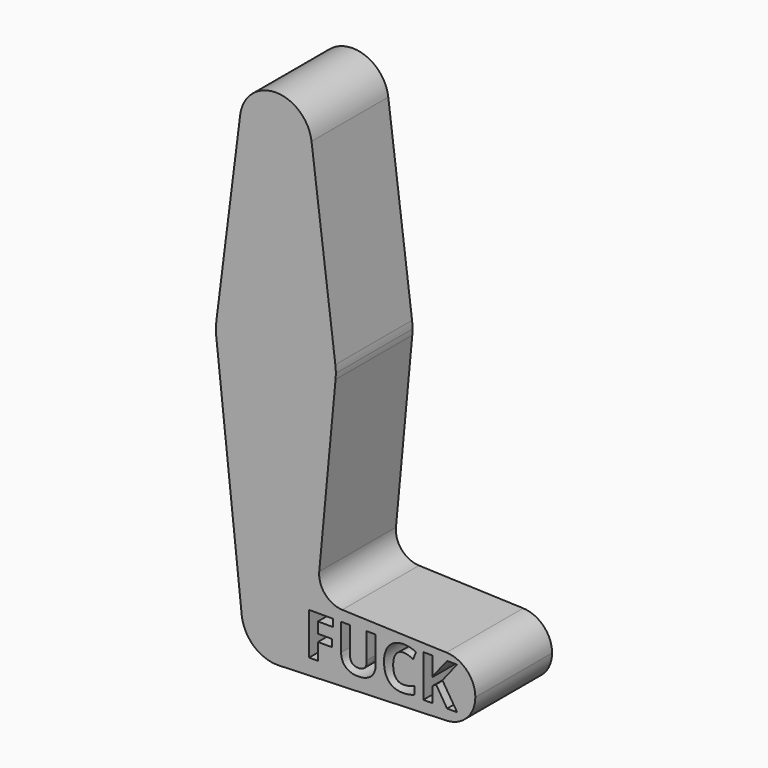
from build123d import *

# Parameters (mm, degrees)
F1_DEPTH     = 25.4
F2_TEXT_SIZE = 15.5810214993
F3_DEPTH     = 25.4


# Not quite as in the source:
# - Text() gives the source's letters only with a copy of the font that has no kerning and outlines rounded to 1/6400 em; it was checked with that copy


with BuildPart() as f1:
    # F0 (on Front) → F1 (new body)
    with BuildSketch(Plane.XZ):
        with BuildLine():
            ThreePointArc((15.8060067394, -1.4784369967), (15.8577423044, -0.7400229765), (15.875, 0))
            ThreePointArc((15.875, 0), (15.8438414904, 0.9941387366), (15.7504882737, 1.984375))
            ThreePointArc((15.7504882737, 1.984375), (0, 15.875), (-15.7504882737, 1.984375))
            ThreePointArc((-15.7504882737, 1.984375), (-15.8743381553, 0.1449590675), (-15.7840999697, -1.6964118445))
            ThreePointArc((-15.7840999697, -1.6964118445), (0.1095364561, -15.8746220983), (15.8060067394, -1.4784369967))
        make_face()
        with BuildLine():
            ThreePointArc((-15.7504882737, 1.984375), (0, 15.875), (15.7504882737, 1.984375))
            Line((15.7504882737, 1.984375), (9.4502929642, 51.990625))
            ThreePointArc((9.4502929642, 51.990625), (9.5063048942, 51.396483242), (9.525, 50.8))
            ThreePointArc((9.525, 50.8), (-0.596483242, 41.2936951058), (-9.4502929642, 51.990625))
            Line((-9.4502929642, 51.990625), (-15.7504882737, 1.984375))
        make_face()
        with BuildLine():
            Line((11.4878163443, -47.6443180191), (15.8060067394, -1.4784369967))
            ThreePointArc((15.8060067394, -1.4784369967), (0.1095364561, -15.8746220983), (-15.7840999697, -1.6964118445))
            Line((-15.7840999697, -1.6964118445), (-9.0323037273, -64.5178471067))
            ThreePointArc((-9.0323037273, -64.5178471067), (-5.7994381843, -70.6984748813), (0.7783348259, -73.0189234444))
            Line((0.7783348259, -73.0189234444), (45.1716383974, -71.4324362036))
            ThreePointArc((45.1716383974, -71.4324362036), (36.9506562545, -63.5), (45.1716383974, -55.5675637964))
            Line((45.1716383974, -55.5675637964), (17.5834333258, -54.5816417807))
            ThreePointArc((17.5834333258, -54.5816417807), (13.0400426858, -52.4271027893), (11.4878163443, -47.6443180191))
        make_face()
        with BuildLine():
            ThreePointArc((9.525, 50.8), (9.5063048942, 51.396483242), (9.4502929642, 51.990625))
            ThreePointArc((9.4502929642, 51.990625), (0, 60.325), (-9.4502929642, 51.990625))
            ThreePointArc((-9.4502929642, 51.990625), (-0.596483242, 41.2936951058), (9.525, 50.8))
        make_face()
        with BuildLine():
            ThreePointArc((52.8256562545, -63.5), (50.6001631592, -57.9884772185), (45.1716383974, -55.5675637964))
            ThreePointArc((45.1716383974, -55.5675637964), (36.9506562545, -63.5), (45.1716383974, -71.4324362036))
            ThreePointArc((45.1716383974, -71.4324362036), (50.6001631592, -69.0115227815), (52.8256562545, -63.5))
        make_face()
    extrude(amount=F1_DEPTH)

    # F2 (on face) → F3 (cut)
    with BuildSketch(Plane.XZ.offset(25.4)):
        with Locations((7.4083339423, -68.5800015926)):
            Text('FUCK', F2_TEXT_SIZE, font='Open Sans', font_style=FontStyle.BOLD, text_align=(TextAlign.LEFT, TextAlign.BOTTOM))
    extrude(amount=-F3_DEPTH, mode=Mode.SUBTRACT)


solid = f1.part
